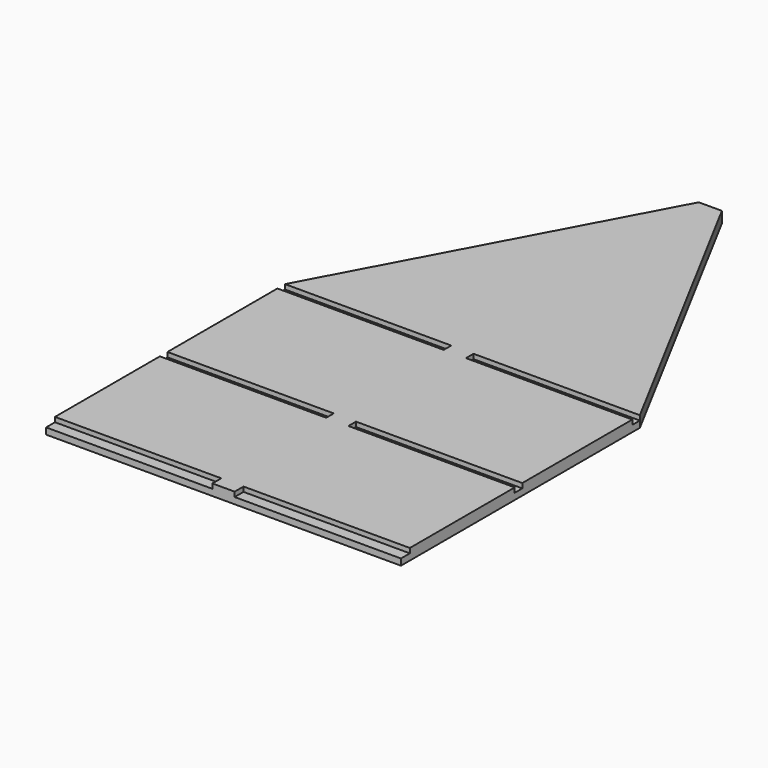
from build123d import *

# Parameters (mm, degrees)
F0_W     = 70.3
F0_H     = 58.1155021116
F1_DEPTH = 4.7
F2_DEPTH = 2.7
F0_H_2   = 4
F0_H_3   = 4.7
F3_DEPTH = 2.7


# Not quite as in the source:
# - a feature names something its author has since deleted; it is built from what else it names


with BuildPart() as f1:
    # F0 (on Top) → F1 (new body)
    with BuildSketch(Plane.XY):
        Polygon((0, -2), (0, 0), (0, 2), (-4.7, 2), (-4.7, -2), (-4.7, -60.1155021116), (-4.7, -64.1155021116), (0, -64.1155021116), (0, -62.1155021116), (0, -60.1155021116), align=None)
        Polygon((0, 2), (0, 0), (0, -2), (0, -60.1155021116), (0, -62.1155021116), (0, -64.1155021116), (4.7, -64.1155021116), (4.7, -60.1155021116), (4.7, -2), (4.7, 2), align=None)
        Polygon((-4.7, 2), (0, 2), (0, 132.9871674252), (-4.9, 132.9871674252), (-75, 2), align=None)
        Polygon((0, 132.9871674252), (0, 2), (4.7, 2), (75, 2), (4.9, 132.9871674252), align=None)
        with Locations((-39.85, -31.0577510558)):
            Rectangle(F0_W, F0_H)
        with Locations((39.85, -31.0577510558)):
            Rectangle(F0_W, F0_H)
        Polygon((4.7, -64.1155021116), (0, -64.1155021116), (0, -124.2310042232), (4.7, -124.2310042232), (4.7, -119.5310042232), (75, -119.5310042232), (75, -64.1155021116), align=None)
        Polygon((0, -124.2310042232), (0, -64.1155021116), (-4.7, -64.1155021116), (-75, -64.1155021116), (-75, -119.5310042232), (-4.7, -119.5310042232), (-4.7, -121.7700988054), (-4.7, -124.2310042232), align=None)
    extrude(amount=F1_DEPTH)

    # F0 (on Top) → F2 (join)
    with BuildSketch(Plane.XY):
        Polygon((-4.7, -2), (-4.7, 2), (-75, 2), (-75, 0), (-75, -2), align=None)
        Polygon((75, 2), (4.7, 2), (4.7, -2), (75, -2), (75, 0), align=None)
    extrude(amount=F2_DEPTH)

    # F0 (on Top) → F3 (join)
    with BuildSketch(Plane.XY):
        with Locations((-39.85, -62.1155021116)):
            Rectangle(F0_W, F0_H_2)
        with Locations((39.85, -62.1155021116)):
            Rectangle(F0_W, F0_H_2)
        Polygon((75, 2), (4.7, 2), (4.7, -2), (75, -2), (75, 0), align=None)
        Polygon((-75, -124.2310042232), (-4.7, -124.2310042232), (-4.7, -121.7700988054), (-4.7, -119.5310042232), (-75, -119.5310042232), align=None)
        with Locations((39.85, -121.8810042232)):
            Rectangle(F0_W, F0_H_3)
    extrude(amount=F3_DEPTH)


solid = f1.part
